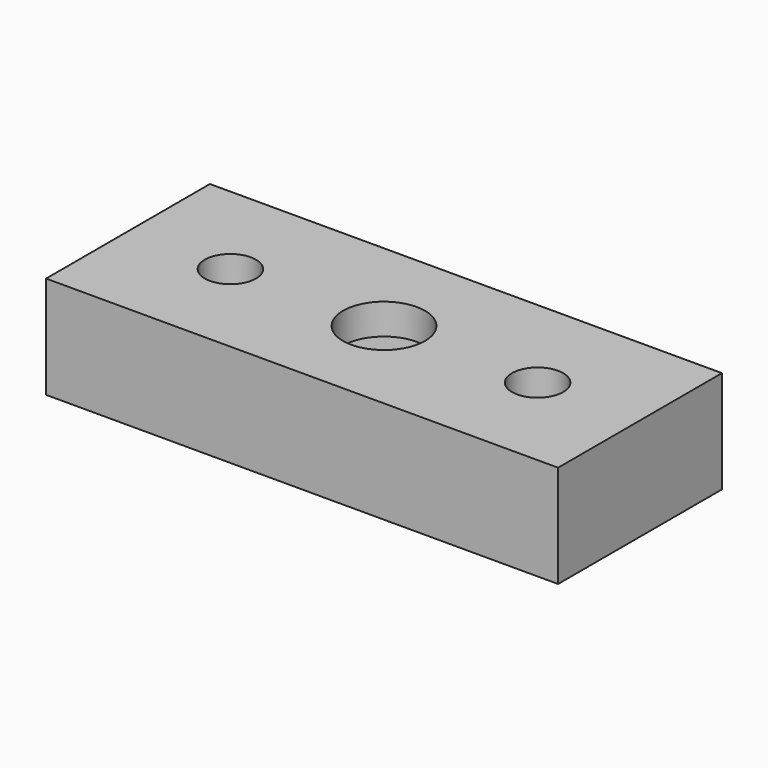
from build123d import *

# Parameters (mm, degrees)
F1_DEPTH = 7
F2_W     = 50
F2_H     = 20
F2_R     = 2.5
F2_R_2   = 4
F3_DEPTH = 3


with BuildPart() as f1:
    # F0 (on Top) → F1 (new body)
    with BuildSketch(Plane.XY):
        with BuildLine():
            Line((25, 0), (25, 10))
            Line((25, 10), (15, 10))
            Line((15, 10), (15, 2.5))
            ThreePointArc((15, 2.5), (16.767767, 1.767767), (17.5, 0))
            Line((17.5, 0), (25, 0))
        make_face()
        with BuildLine():
            Line((15, 2.5), (15, 10))
            Line((15, 10), (-15, 10))
            Line((-15, 10), (-15, 2.5))
            ThreePointArc((-15, 2.5), (-13.232233, 1.767767), (-12.5, 0))
            ThreePointArc((-12.5, 0), (-15, -2.5), (-17.5, 0))
            Line((-17.5, 0), (-25, 0))
            Line((-25, 0), (-25, -10))
            Line((-25, -10), (25, -10))
            Line((25, -10), (25, 0))
            Line((25, 0), (17.5, 0))
            ThreePointArc((17.5, 0), (13.232233, -1.767767), (15, 2.5))
        make_face()
        Polygon((0, 7.390083), (6.4, 3.695042), (6.4, -3.695042), (0, -7.390083), (-6.4, -3.695042), (-6.4, 3.695042), align=None, mode=Mode.SUBTRACT)
        with BuildLine():
            Line((-15, 2.5), (-15, 10))
            Line((-15, 10), (-25, 10))
            Line((-25, 10), (-25, 0))
            Line((-25, 0), (-17.5, 0))
            ThreePointArc((-17.5, 0), (-16.767767, 1.767767), (-15, 2.5))
        make_face()
    extrude(amount=F1_DEPTH)

    # F2 (on face) → F3 (join)
    with BuildSketch(Plane.XY.offset(7)):
        Rectangle(F2_W, F2_H)
        with Locations((-15, 0)):
            Circle(F2_R, mode=Mode.SUBTRACT)
        Polygon((0, -7.390083), (-6.4, -3.695042), (-6.4, 3.695042), (0, 7.390083), (6.4, 3.695042), (6.4, -3.695042), align=None, mode=Mode.SUBTRACT)
        with Locations((15, 0)):
            Circle(F2_R, mode=Mode.SUBTRACT)
        Polygon((-6.4, 3.695042), (-6.4, -3.695042), (0, -7.390083), (6.4, -3.695042), (6.4, 3.695042), (0, 7.390083), align=None)
        Circle(F2_R_2, mode=Mode.SUBTRACT)
    extrude(amount=F3_DEPTH)


solid = f1.part
